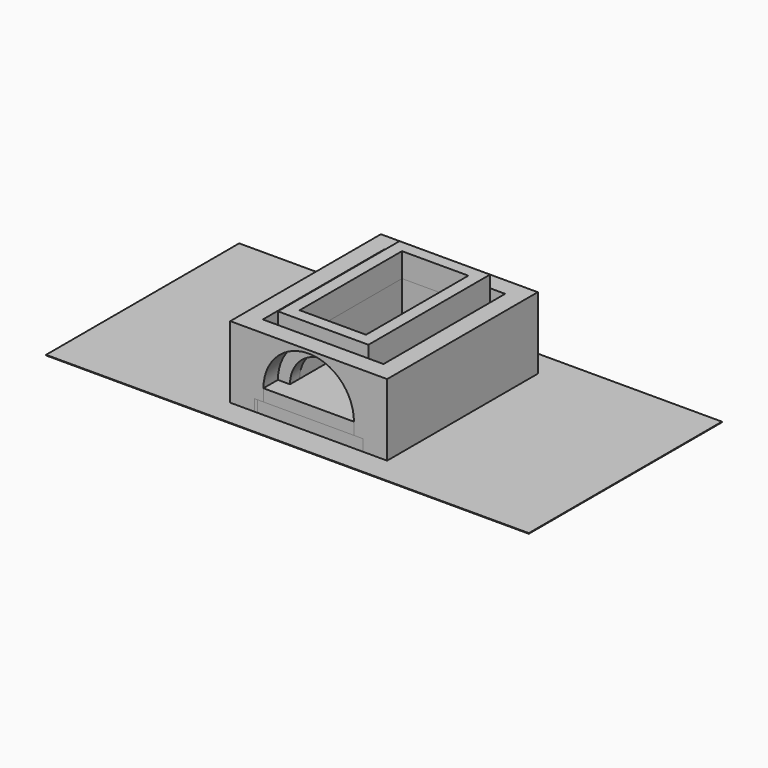
from build123d import *

# Parameters (mm, degrees)
F0_W      = 1300
F0_H      = 1560
F1_DEPTH  = 200
F2_W      = 1300
F2_H      = 1560
F2_W_2    = 1000
F2_H_2    = 1260
F3_DEPTH  = 600
F5_DEPTH  = 150
F6_W      = 750
F6_H      = 1260
F6_W_2    = 550
F6_H_2    = 1060
F7_DEPTH  = 700
F9_DEPTH  = 100
F10_W     = 900
F10_H     = 1560
F11_DEPTH = 100
F12_SIZE  = 25
F13_W     = 750
F13_H     = 1260
F13_W_2   = 550
F13_H_2   = 1060
F14_DEPTH = 500
F16_DEPTH = 100
F17_W     = 900
F17_H     = 1560
F18_DEPTH = 100
F19_SIZE  = 25
F20_W     = 4000
F20_H     = 2000
F21_DEPTH = 5


with BuildPart() as f1:
    # F0 (on Top) → F1 (new body)
    with BuildSketch(Plane.XY):
        Rectangle(F0_W, F0_H)
    extrude(amount=F1_DEPTH)


with BuildPart() as f3:
    # F2 (on Top) → F3 (new body)
    with BuildSketch(Plane.XY):
        Rectangle(F2_W, F2_H)
        Rectangle(F2_W_2, F2_H_2, mode=Mode.SUBTRACT)
    extrude(amount=F3_DEPTH)

    # F4 (on face) → F5 (cut, through all)
    with BuildSketch(Plane.XZ.offset(780)):
        with BuildLine():
            Line((-375, 200), (-375, 0))
            Line((-375, 0), (375, 0))
            Line((375, 0), (375, 200))
            ThreePointArc((375, 200), (0, 575), (-375, 200))
        make_face()
    extrude(amount=-F5_DEPTH, mode=Mode.SUBTRACT)


with BuildPart() as f7:
    # F6 (on Top) → F7 (new body)
    with BuildSketch(Plane.XY):
        Rectangle(F6_W, F6_H)
        Rectangle(F6_W_2, F6_H_2, mode=Mode.SUBTRACT)
    extrude(amount=F7_DEPTH)

    # F8 (on face) → F9 (cut, through all)
    with BuildSketch(Plane.XZ.offset(630)):
        with BuildLine():
            Line((-275, 300), (-275, 0))
            Line((-275, 0), (275, 0))
            Line((275, 0), (275, 300))
            ThreePointArc((275, 300), (0, 575), (-275, 300))
        make_face()
    extrude(amount=-F9_DEPTH, mode=Mode.SUBTRACT)


with BuildPart() as f11:
    # F10 (on Top) → F11 (new body)
    with BuildSketch(Plane.XY):
        Rectangle(F10_W, F10_H)
    extrude(amount=F11_DEPTH)

    # F12
    f12_edges = [f11.edges().sort_by_distance(p)[0] for p in [
        (450, -780, 50),
        (450, 780, 50),
    ]]
    chamfer(f12_edges, length=F12_SIZE)


with BuildPart() as f14:
    # F13 (on Top) → F14 (new body)
    with BuildSketch(Plane.XY):
        Rectangle(F13_W, F13_H)
        Rectangle(F13_W_2, F13_H_2, mode=Mode.SUBTRACT)
    extrude(amount=F14_DEPTH)

    # F15 (on face) → F16 (cut, through all)
    with BuildSketch(Plane.XZ.offset(630)):
        with BuildLine():
            Line((-275, 200), (-275, 0))
            Line((-275, 0), (275, 0))
            Line((275, 0), (275, 200))
            ThreePointArc((275, 200), (0, 475), (-275, 200))
        make_face()
    extrude(amount=-F16_DEPTH, mode=Mode.SUBTRACT)


with BuildPart() as f18:
    # F17 (on Top) → F18 (new body)
    with BuildSketch(Plane.XY):
        Rectangle(F17_W, F17_H)
    extrude(amount=F18_DEPTH)

    # F19
    f19_edges = [f18.edges().sort_by_distance(p)[0] for p in [
        (-450, -780, 50),
        (-450, 780, 50),
    ]]
    chamfer(f19_edges, length=F19_SIZE)


with BuildPart() as f21:
    # F20 (on Top) → F21 (new body)
    with BuildSketch(Plane.XY):
        Rectangle(F20_W, F20_H)
    extrude(amount=F21_DEPTH)


solid = Compound([f1.part, f3.part, f7.part, f11.part, f14.part, f18.part, f21.part])
